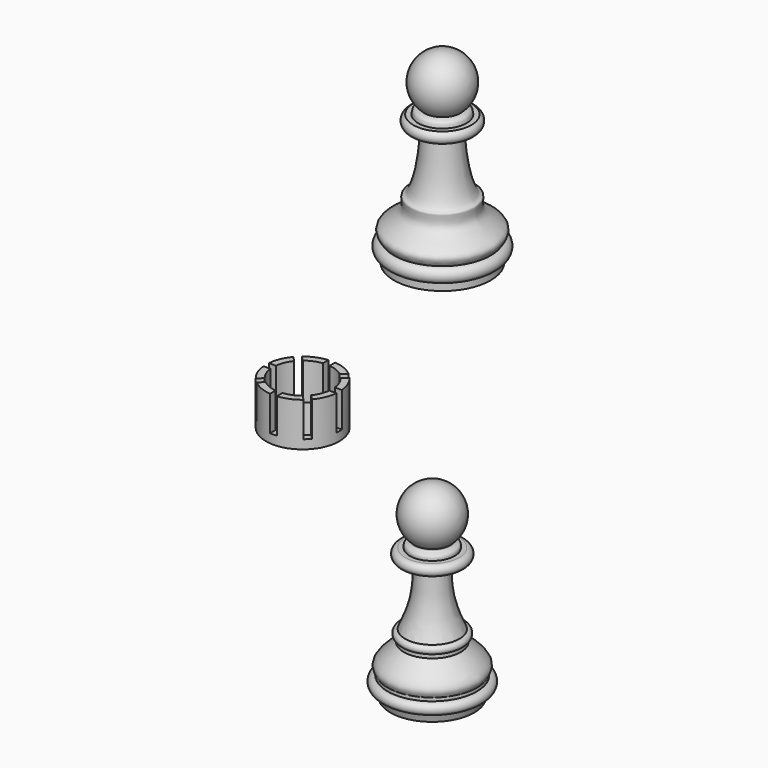
from build123d import *

# Parameters (mm, degrees)
F0_W            = 6.6979378462
F0_H            = 7.9824775457
F4_T            = -1.27
F6_DEPTH        = 6.35
F6_COPIES_COUNT = 8


# Not quite as in the source:
# - a pattern or mirror of a feature is missing from the dataset's text; its kind, count and spacing are read off the source's solid


with BuildPart() as f1:
    # F0 (on Front) → F1 (revolve)
    with BuildSketch(Plane.XZ):
        with BuildLine():
            add(Edge.make_bspline(
                [(148.7789601088, -38.950316608), (149.1387025112, -39.0406037985), (149.8345363416, -39.2152423209), (149.894497256, -39.8677474324), (149.9234586954, -40.1829108596)],
                knots=[0, 0, 0, 0, 0.5169947, 1, 1, 1, 1], degree=3))
            ThreePointArc((148.7789601088, -38.950316608), (150.3347219752, -33.2591866073), (145.5074697733, -29.8669908807))
            Line((145.5074697733, -29.8669908807), (145.5074697733, -64.0146881342))
            Line((145.5074697733, -64.0146881342), (154.3417721987, -64.0146881342))
            Line((154.3417721987, -64.0146881342), (154.3417721987, -62.6460984349))
            ThreePointArc((154.3417721987, -62.6460984349), (155.504018215, -61.3330155611), (154.3417721987, -60.0199326873))
            add(Edge.make_bspline(
                [(148.597612977, -42.1716943383), (148.8047871619, -44.7013404483), (149.1587242701, -49.0229967844), (150.5485886489, -53.092426934), (151.6866239156, -53.0357410053), (150.5037728043, -55.9815689857), (155.8212260112, -57.9147702783), (154.7573833416, -59.428546226), (154.3417721987, -60.0199326873)],
                knots=[0, 0, 0, 0, 0.263046792, 0.4493900673, 0.5225636147, 0.6648557255, 0.8690692722, 1, 1, 1, 1], degree=3))
            Line((148.597612977, -42.1716943383), (150.8216261864, -42.1716943383))
            ThreePointArc((150.8216261864, -42.1716943383), (151.4850268973, -41.177302599), (150.8216261864, -40.1829108596))
            Line((150.8216261864, -40.1829108596), (149.9234586954, -40.1829108596))
        make_face()
    revolve(axis=Axis((145.5074697733, 0, -46.9408395074), (0, 0, -1)))


with BuildPart() as f2:
    # F0 (on Front) → F2 (revolve)
    with BuildSketch(Plane.XZ):
        with BuildLine():
            add(Edge.make_bspline(
                [(146.8999534845, -109.0292558074), (146.8576441295, -109.1695647974), (146.7548941379, -109.5103108935), (147.7896890033, -109.5723780868), (147.7713317923, -110.1745251961), (147.7620452642, -110.4791387916)],
                knots=[0, 0, 0, 0, 0.2569983953, 0.624131069, 1, 1, 1, 1], degree=3))
            ThreePointArc((146.8999534845, -109.0292558074), (148.4736204885, -103.3618111947), (143.6656713486, -99.9735990784))
            Line((143.6656713486, -99.9735990784), (143.6656713486, -109.0292558074))
            Line((143.6656713486, -109.0292558074), (143.6656713486, -134.5115453005))
            Line((143.6656713486, -134.5115453005), (151.3320356607, -134.5115453005))
            Line((151.3320356607, -134.5115453005), (151.8040299416, -132.9853236675))
            ThreePointArc((151.8040299416, -132.9853236675), (152.9242608777, -131.9707110524), (151.8040299416, -130.9560984373))
            Line((151.8040299416, -130.9560984373), (151.8040299416, -130.3542852402))
            add(Edge.make_bspline(
                [(148.863479495, -125.5910694599), (150.4008443737, -126.8625837497), (152.7504184668, -128.8058550418), (152.0471413144, -129.9565194376), (151.8040299416, -130.3542852402)],
                knots=[0, 0, 0, 0, 0.6543164071, 1, 1, 1, 1], degree=3))
            Line((148.863479495, -125.5910694599), (148.863479495, -124.910607934))
            ThreePointArc((148.863479495, -124.910607934), (149.3645873733, -124.1106469588), (148.6154645681, -123.53631109))
            add(Edge.make_bspline(
                [(146.3153958321, -112.4079972506), (146.3937953533, -114.5733581792), (146.5432129123, -118.7002066468), (147.9478444177, -121.9782567066), (148.6154645681, -123.53631109)],
                knots=[0, 0, 0, 0, 0.5247008572, 1, 1, 1, 1], degree=3))
            Line((146.3153958321, -112.4079972506), (148.5914587975, -112.4079972506))
            ThreePointArc((148.5914587975, -112.4079972506), (149.555888027, -111.4435680211), (148.5914587975, -110.4791387916))
            Line((148.5914587975, -110.4791387916), (147.7620452642, -110.4791387916))
        make_face()
    revolve(axis=Axis((143.6656713486, 0, -121.7704005539), (0, 0, -1)))


with BuildPart() as f3:
    # F0 (on Front) → F3 (revolve)
    with BuildSketch(Plane.XZ):
        with Locations((123.3333721757, -94.9059799314)):
            Rectangle(F0_W, F0_H)
    revolve(axis=Axis((119.9844032526, 0, -94.9059799314), (0, 0, -1)))

    # F4
    f4_openings = [f3.faces().sort_by_distance(p)[0] for p in [
        (119.984403, 0, -90.914741),
    ]]
    offset(amount=F4_T, openings=f4_openings)

    # F5 (on face) → F6 (cut)
    with BuildSketch(Plane.XY.offset(-90.9147411585)):
        with BuildLine():
            Line((120.5996051431, 5.3929616998), (120.5996051431, 6.6696250288))
            ThreePointArc((120.5996051431, 6.6696250288), (119.9844032526, 6.6979378462), (119.3692013621, 6.6696250288))
            Line((119.3692013621, 6.6696250288), (119.3692013621, 5.3929616998))
            ThreePointArc((119.3692013621, 5.3929616998), (119.9844032526, 5.4279378462), (120.5996051431, 5.3929616998))
        make_face()
    f6 = extrude(amount=-F6_DEPTH, mode=Mode.SUBTRACT)

    # F6_copies: F6 ×8 about axis
    f6_copies_axis = Axis((119.984403, 0, 0), (0, 0, 1))
    for i in range(1, F6_COPIES_COUNT):
        add(f6.rotate(f6_copies_axis, i * 360 / F6_COPIES_COUNT), mode=Mode.SUBTRACT)


solid = Compound([f1.part, f2.part, f3.part])
